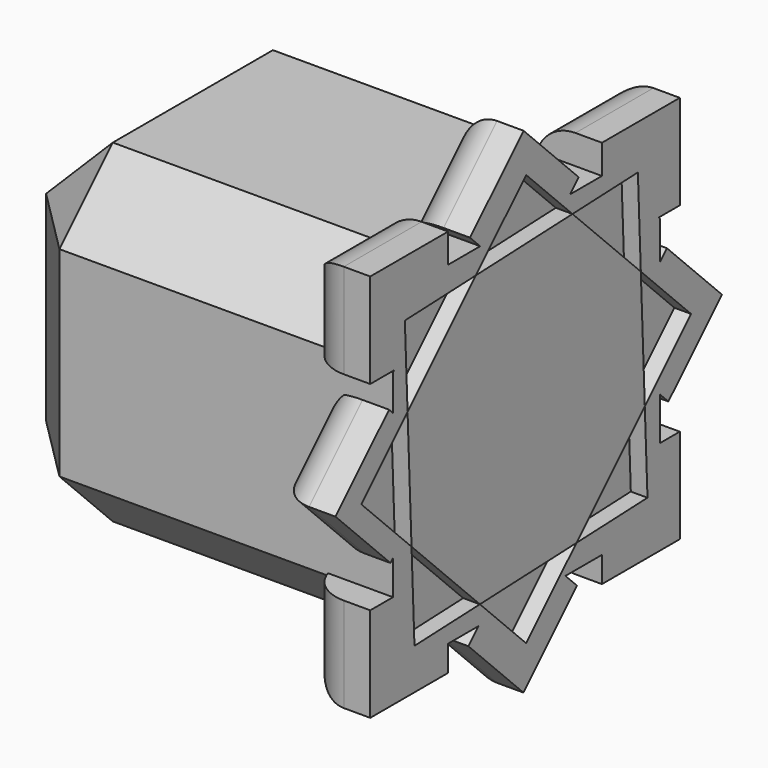
from build123d import *

# Parameters (mm, degrees)
F0_W       = 25.4
F0_H       = 25.4
F1_DEPTH   = 25.4
F2_W       = 5.2458834782
F2_H       = 4.983584857
F2_W_2     = 5.5085764325
F2_H_2     = 5.2462833226
F1_FACE_W  = 25.4
F1_FACE_H  = 25.4
F1_FACE1_W = 25.4
F1_FACE1_H = 25.4
F3_DEPTH   = 2.54
F5_DEPTH   = 5.08
F6_SIZE    = 5.08
F7_R       = 3.0660512242
F9_DEPTH   = 1.27
F10_DEPTH  = 9.652


# Not quite as in the source:
# - a feature names something its author has since deleted; it is built from what else it names


with BuildPart() as f1:
    # F0 (on Front) → F1 (new body)
    with BuildSketch(Plane.XZ):
        Rectangle(F0_W, F0_H)
    extrude(amount=F1_DEPTH)

    # F2 (on face) + F1_face (on face) + F1_face1 (on face) → F3 (join, symmetric)
    with BuildSketch(Plane.YZ.offset(12.7)):
        Polygon((-27.5641178384, 14.9262829959), (-27.5641178384, 7.716415143), (-25.4, 7.716415143), (-25.4, 12.7), (-20.1541165218, 12.7), (-20.1541165218, 14.9262829959), align=None)
        with Locations((-22.7770582609, 10.2082075715)):
            Rectangle(F2_W, F2_H)
        with Locations((-2.7542882162, 10.2082075715)):
            Rectangle(F2_W_2, F2_H)
        Polygon((-5.5085764325, 14.9262829959), (-5.5085764325, 12.7), (0, 12.7), (0, 7.716415143), (1.9014248842, 7.716415143), (1.9014248842, 14.9262829959), align=None)
        Polygon((0, -12.7), (-5.5085764325, -12.7), (-5.5085764325, -14.6635845304), (1.9014248842, -14.6635845304), (1.9014248842, -7.4537166774), (0, -7.4537166774), align=None)
        Polygon((-25.4, -12.7), (-25.4, -7.4537166774), (-27.5641178384, -7.4537166774), (-27.5641178384, -14.6635845304), (-20.1541165218, -14.6635845304), (-20.1541165218, -12.7), align=None)
        with Locations((-2.7542882162, -10.0768583387)):
            Rectangle(F2_W_2, F2_H_2)
    with BuildSketch(Plane(origin=(12.7, -12.7, 0), x_dir=(0, 1, 0), z_dir=(1, 0, 0))):
        Rectangle(F1_FACE_W, F1_FACE_H)
    with BuildSketch(Plane(origin=(-12.7, -12.7, 0), x_dir=(0, -1, 0), z_dir=(-1, 0, 0))):
        Rectangle(F1_FACE1_W, F1_FACE1_H)
    extrude(amount=F3_DEPTH, both=True, dir=(1, 0, 0))

    # F4 (on face) → F5 (join)
    with BuildSketch(Plane.YZ.offset(15.24)):
        Polygon((-12.9697233272, 18.7644396144), (-18.0678697774, 13.6662931641), (-17.1015766133, 12.7), (-8.5548385823, 12.7), (-7.7300611476, 13.5247774348), align=None)
        Polygon((0.6718987712, 5.3462631056), (0, 4.6743643344), (0, -4.1781310237), (0.8134145006, -4.9915455243), (5.9115609509, 0.106600926), align=None)
        Polygon((-8.9828089794, -12.7), (-17.2593100241, -12.7), (-18.219205952, -13.6598959279), (-12.9795437724, -18.8995581075), (-7.8813973221, -13.8014116573), align=None)
        Polygon((-25.4, -4.8368342047), (-25.4, 4.8952218766), (-25.773634139, 5.2688560155), (-30.8717805892, 0.1707095653), (-25.6321184096, -5.0689526143), align=None)
    extrude(amount=-F5_DEPTH)

    # F6
    f6_edges = [f1.edges().sort_by_distance(p)[0] for p in [
        (-2.54, 0, -12.7),
        (-15.24, 0, 0),
        (-15.24, -12.7, 12.7),
        (-15.24, -12.7, -12.7),
        (-15.24, -25.4, 0),
        (-2.54, -25.4, 12.7),
        (-2.54, -25.4, -12.7),
        (-2.54, 0, 12.7),
    ]]
    chamfer(f6_edges, length=F6_SIZE)

    # F7
    f7_edges = [f1.edges().sort_by_distance(p)[0] for p in [
        (10.16, -15.599375, -16.279727),
        (10.16, -10.430471, -16.350485),
        (10.16, -1.803576, -14.663585),
        (10.16, 1.901425, -11.058651),
        (10.16, -23.859117, -14.663585),
        (10.16, -27.564118, -11.058651),
        (10.16, -28.251949, -2.449122),
        (10.16, -28.322707, 2.719783),
        (10.16, -27.564118, 11.321349),
        (10.16, -23.859117, 14.926283),
        (10.16, 3.362488, -2.442472),
        (10.16, 3.29173, 2.726432),
        (10.16, 1.901425, 11.321349),
        (10.16, -1.803576, 14.926283),
        (10.16, -10.349892, 16.144609),
        (10.16, -15.518797, 16.215366),
    ]]
    fillet(f7_edges, radius=F7_R)

    # F8 (on face) → F9 (cut)
    with BuildSketch(Plane.YZ.offset(15.24)):
        Polygon((-1.4303888491, -4.4065409636), (2.9761521146, 0), (-1.8094554409, 4.7856075555), align=None)
        Polygon((-1.1736200056, -10.6330388789), (-1.4303888491, -4.4065409636), (-7.9357437924, -10.911895907), align=None)
        Polygon((-7.9357437924, -10.911895907), (-1.4303888491, -4.4065409636), (-1.8094554409, 4.7856075555), (-8.3148103842, 11.2909624988), (-17.5069589033, 10.911895907), (-24.0123138467, 4.4065409636), (-23.6332472548, -4.7856075555), (-17.1278923115, -11.2909624988), align=None)
        Polygon((-8.3148103842, 11.2909624988), (-1.8094554409, 4.7856075555), (-2.0883124689, 11.5477313422), align=None)
        Polygon((-12.7213513479, -15.6975034624), (-7.9357437924, -10.911895907), (-17.1278923115, -11.2909624988), align=None)
        Polygon((-17.5069589033, 10.911895907), (-8.3148103842, 11.2909624988), (-12.7213513479, 15.6975034624), align=None)
        Polygon((-23.3543902268, -11.5477313422), (-17.1278923115, -11.2909624988), (-23.6332472548, -4.7856075555), align=None)
        Polygon((-24.0123138467, 4.4065409636), (-17.5069589033, 10.911895907), (-24.2690826901, 10.6330388789), align=None)
        Polygon((-28.4188548103, 0), (-23.6332472548, -4.7856075555), (-24.0123138467, 4.4065409636), align=None)
    extrude(amount=-F9_DEPTH, mode=Mode.SUBTRACT)


with BuildPart() as f10:
    # F8 (on face) → F10 (new body)
    with BuildSketch(Plane.YZ.offset(15.24)):
        Polygon((-7.9357437924, -10.911895907), (-1.4303888491, -4.4065409636), (-1.8094554409, 4.7856075555), (-8.3148103842, 11.2909624988), (-17.5069589033, 10.911895907), (-24.0123138467, 4.4065409636), (-23.6332472548, -4.7856075555), (-17.1278923115, -11.2909624988), align=None)
    extrude(amount=-F10_DEPTH)


solid = Compound([f1.part, f10.part])
